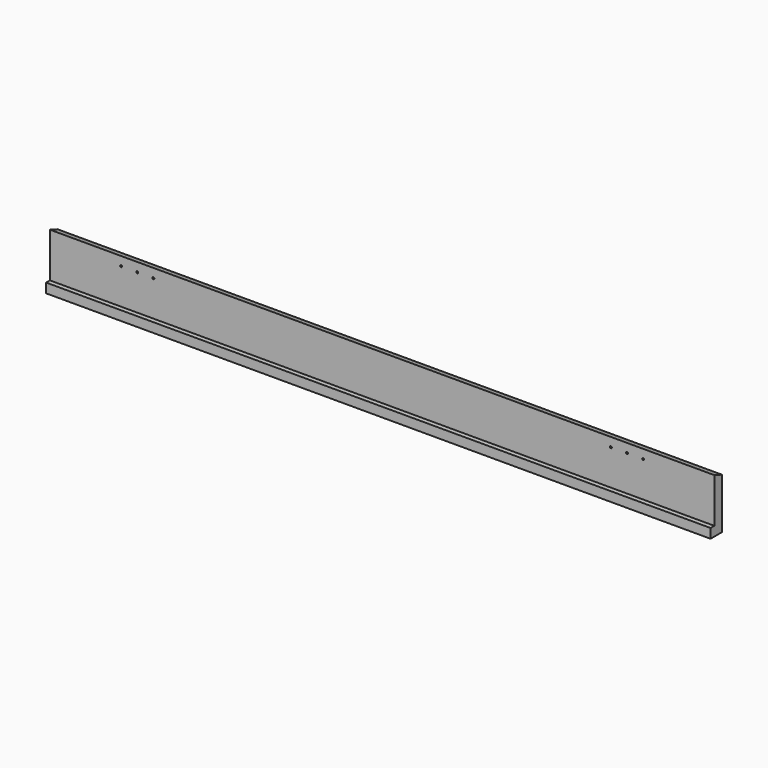
from build123d import *

# Parameters (mm, degrees)
F1_DEPTH = 70
F2_SIZE2 = 0.36396
F2_SIZE  = 0.99999
F4_D     = 0.2
F4_DEPTH = 0.9
F4_TIP   = 0.0600860619


# Not quite as in the source:
# - a fillet or chamfer is up to 0.001 mm smaller than in the source, because OpenCascade refuses the exact size


with BuildPart() as f1:
    # F0 (on Right) → F1 (new body)
    with BuildSketch(Plane.YZ):
        Polygon((-39.5598503354, -13.8284793004), (-40.5598503354, -13.8284793004), (-40.5598503354, -18.5284793004), (-41.0598503354, -18.5284793004), (-41.0598503354, -19.5284793004), (-39.5598503354, -19.5284793004), align=None)
    extrude(amount=-F1_DEPTH)

    # F2 (size 1 and 0.3639702343 in the source; OpenCascade refuses exactly that, so slightly less here)
    f2_edges = [f1.edges().sort_by_distance(p)[0] for p in [
        (-35, -39.55985, -13.828479),
    ]]
    f2_side = f1.faces().sort_by_distance((-35, -40.05985, -13.828479))[0]
    chamfer(f2_edges, length=F2_SIZE, length2=F2_SIZE2, reference=f2_side)

    # F4
    with Locations(Plane.XZ.offset(40.5598503354)):
        with Locations((-62.5, -14.7784793004), (-60.8, -14.7784793004), (-59.1, -14.7784793004), (-10.9, -14.7784793004), (-9.2, -14.7784793004), (-7.5, -14.7784793004)):
            Hole(F4_D / 2, depth=F4_DEPTH)
            with Locations((0, 0, -(F4_DEPTH + F4_TIP / 2))):  # 118° drill point
                Cone(0, F4_D / 2, F4_TIP, mode=Mode.SUBTRACT)


solid = f1.part
